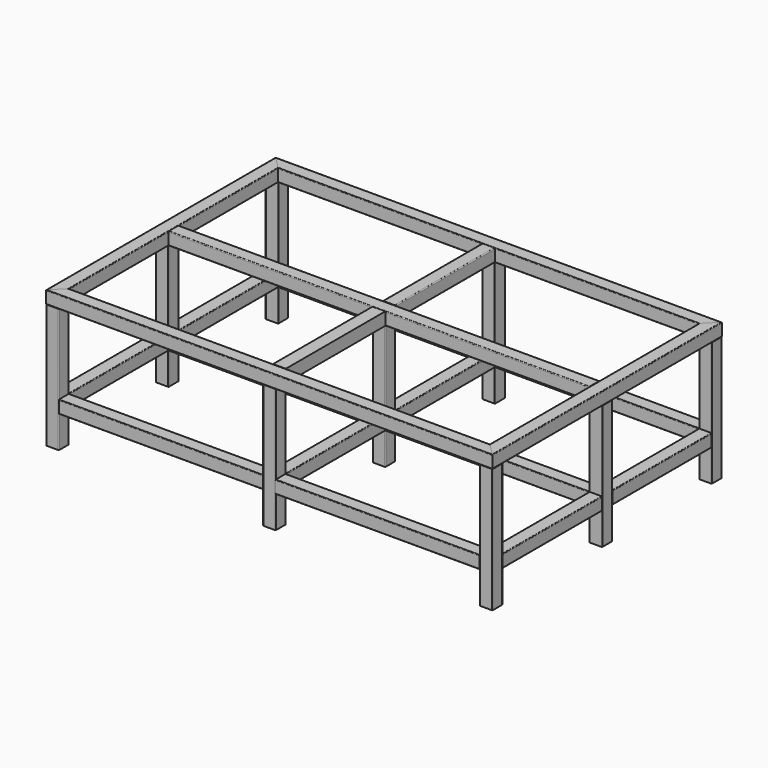
from build123d import *

# Parameters (mm, degrees)
F1_DEPTH  = 80
F2_W      = 70
F2_H      = 70
F3_DEPTH  = 1000
F4_R      = 4
F5_R      = 4
F7_DEPTH  = 80
F8_W      = 70
F8_H      = 70
F9_DEPTH  = 1400
F10_R     = 4
F11_R     = 4
F12_W     = 2640
F12_H     = 80
F13_DEPTH = 80
F14_W     = 70
F14_H     = 70
F15_DEPTH = 2640
F16_R     = 5
F17_W     = 80
F17_H     = 780
F18_DEPTH = 80
F19_W     = 70
F19_H     = 70
F20_DEPTH = 1560
F21_W     = 70
F21_H     = 70
F22_DEPTH = 1640
F23_R     = 5
F24_W     = 3000
F24_H     = 2000
F25_DEPTH = 60
F27_DEPTH = 780
F28_W     = 1280
F28_H     = 80
F29_DEPTH = 80
F31_DEPTH = 1280
F32_R     = 4
F34_DEPTH = 1280
F35_R     = 4
F36_W     = 1280
F36_H     = 80
F37_DEPTH = 80
F38_W     = 1280
F38_H     = 80
F39_DEPTH = 80
F41_DEPTH = 1280
F42_R     = 4
F42_2_R   = 4
F44_DEPTH = 1280
F45_R     = 4
F46_R     = 4
F47_W     = 780
F47_H     = 80
F48_DEPTH = 80
F49_W     = 780
F49_H     = 80
F50_DEPTH = 80
F51_W     = 780
F51_H     = 80
F52_DEPTH = 80
F54_DEPTH = 780
F55_R     = 4
F55_2_R   = 4
F55_3_R   = 4
F57_DEPTH = 780
F58_R     = 4
F58_2_R   = 4
F58_3_R   = 4


with BuildPart() as f1:
    # F0 (on Top) → F1 (new body)
    with BuildSketch(Plane.XY):
        Polygon((-1400, 900), (-1400, -900), (-1320, -820), (-1320, 820), align=None)
    extrude(amount=F1_DEPTH)


with BuildPart() as f1b:
    # F0 (on Top) → F1, piece 2 (new body)
    with BuildSketch(Plane.XY):
        Polygon((1320, 820), (1320, -820), (1400, -900), (1400, 900), align=None)
    extrude(amount=F1_DEPTH)


with BuildPart() as f3_tool:
    # F2 (on Front) → F3 (new body, symmetric)
    with BuildSketch(Plane.XZ):
        with Locations((-1360, 40)):
            Rectangle(F2_W, F2_H)
        with Locations((1360, 40)):
            Rectangle(F2_W, F2_H)
    extrude(amount=F3_DEPTH, both=True)


with BuildPart() as f1_1:
    add(f1.part)

    # F3: cut by f3_tool
    add(f3_tool.part, mode=Mode.SUBTRACT)

    # F4
    f4_edges = [f1_1.edges().sort_by_distance(p)[0] for p in [
        (-1400, 0, 80),
        (-1320, 0, 80),
        (-1320, 0, 0),
        (-1400, 0, 0),
        (-1325, 0, 75),
        (-1395, 0, 75),
        (-1325, 0, 5),
        (-1395, 0, 5),
    ]]
    fillet(f4_edges, radius=F4_R)


with BuildPart() as f1b_1:
    add(f1b.part)

    # F3: cut by f3_tool
    add(f3_tool.part, mode=Mode.SUBTRACT)

    # F5
    f5_edges = [f1b_1.edges().sort_by_distance(p)[0] for p in [
        (1400, 0, 80),
        (1400, 0, 0),
        (1320, 0, 80),
        (1320, 0, 0),
        (1395, 0, 75),
        (1395, 0, 5),
        (1325, 0, 5),
        (1325, 0, 75),
    ]]
    fillet(f5_edges, radius=F5_R)


with BuildPart() as f7:
    # F6 (on Top) → F7 (new body)
    with BuildSketch(Plane.XY):
        Polygon((1320, -820), (-1320, -820), (-1400, -900), (1400, -900), align=None)
    extrude(amount=F7_DEPTH)


with BuildPart() as f7b:
    # F6 (on Top) → F7, piece 2 (new body)
    with BuildSketch(Plane.XY):
        Polygon((1400, 900), (-1400, 900), (-1320, 820), (1320, 820), align=None)
    extrude(amount=F7_DEPTH)


with BuildPart() as f9_tool:
    # F8 (on Right) → F9 (new body, symmetric)
    with BuildSketch(Plane.YZ):
        with Locations((-860, 40)):
            Rectangle(F8_W, F8_H)
        with Locations((860, 40)):
            Rectangle(F8_W, F8_H)
    extrude(amount=F9_DEPTH, both=True)


with BuildPart() as f7_1:
    add(f7.part)

    # F9: cut by f9_tool
    add(f9_tool.part, mode=Mode.SUBTRACT)

    # F10
    f10_edges = [f7_1.edges().sort_by_distance(p)[0] for p in [
        (0, -900, 0),
        (0, -820, 0),
        (0, -820, 80),
        (0, -900, 80),
        (0, -895, 5),
        (0, -825, 5),
        (0, -825, 75),
        (0, -895, 75),
    ]]
    fillet(f10_edges, radius=F10_R)


with BuildPart() as f7b_1:
    add(f7b.part)

    # F9: cut by f9_tool
    add(f9_tool.part, mode=Mode.SUBTRACT)

    # F11
    f11_edges = [f7b_1.edges().sort_by_distance(p)[0] for p in [
        (0, 820, 80),
        (0, 900, 80),
        (0, 820, 0),
        (0, 895, 5),
        (0, 895, 75),
        (0, 900, 0),
        (0, 825, 75),
        (0, 825, 5),
    ]]
    fillet(f11_edges, radius=F11_R)


with BuildPart() as f13:
    # F12 (on Top) → F13 (new body)
    with BuildSketch(Plane.XY):
        Rectangle(F12_W, F12_H)
    extrude(amount=F13_DEPTH)

    # F14 (on face) → F15 (cut)
    with BuildSketch(Plane(origin=(-1320, 0, 0), x_dir=(0, -1, 0), z_dir=(-1, 0, 0))):
        with Locations((0, 40)):
            Rectangle(F14_W, F14_H)
    extrude(amount=-F15_DEPTH, mode=Mode.SUBTRACT)

    # F16
    f16_edges = [f13.edges().sort_by_distance(p)[0] for p in [
        (0, -40, 0),
        (0, 40, 0),
        (0, 40, 80),
        (0, -35, 75),
        (0, -40, 80),
        (0, -35, 5),
        (0, 35, 5),
        (0, 35, 75),
    ]]
    fillet(f16_edges, radius=F16_R)


with BuildPart() as f18:
    # F17 (on Top) → F18 (new body)
    with BuildSketch(Plane.XY):
        with Locations((0, 430)):
            Rectangle(F17_W, F17_H)
    extrude(amount=F18_DEPTH)


with BuildPart() as f18b:
    # F17 (on Top) → F18, piece 2 (new body)
    with BuildSketch(Plane.XY):
        with Locations((0, -430)):
            Rectangle(F17_W, F17_H)
    extrude(amount=F18_DEPTH)


with BuildPart() as f20_tool:
    # F19 (on face) → F20 (new body)
    with BuildSketch(Plane.XZ.offset(820)):
        with Locations((0, 40)):
            Rectangle(F19_W, F19_H)
    extrude(amount=-F20_DEPTH)


with BuildPart() as f18_1:
    add(f18.part)

    # F20: cut by f20_tool
    add(f20_tool.part, mode=Mode.SUBTRACT)

    # F21 (on face) → F22 (cut)
    with BuildSketch(Plane(origin=(0, 820, 0), x_dir=(-1, 0, 0), z_dir=(0, 1, 0))):
        with Locations((0, 40)):
            Rectangle(F21_W, F21_H)
    extrude(amount=-F22_DEPTH, mode=Mode.SUBTRACT)

    # F23
    f23_edges = [f18_1.edges().sort_by_distance(p)[0] for p in [
        (40, 430, 80),
        (-40, 430, 80),
        (40, 430, 0),
        (-40, 430, 0),
        (35, 430, 75),
        (35, 430, 5),
        (-35, 430, 5),
        (-35, 430, 75),
    ]]
    fillet(f23_edges, radius=F23_R)


with BuildPart() as f18b_1:
    add(f18b.part)

    # F20: cut by f20_tool
    add(f20_tool.part, mode=Mode.SUBTRACT)


with BuildPart() as f25:
    # F24 (on face) → F25 (new body)
    with BuildSketch(Plane.XY.offset(80)):
        Rectangle(F24_W, F24_H)
    extrude(amount=F25_DEPTH)


with BuildPart() as f27:
    # F26 (on face) → F27 (new body)
    with BuildSketch(Plane(origin=(0, 0, 0), x_dir=(1, 0, 0), z_dir=(0, 0, -1))):
        with BuildLine():
            Line((1324, -900), (1396, -900))
            ThreePointArc((1396, -900), (1398.8284271247, -898.8284271247), (1400, -896))
            Line((1400, -896), (1400, -824))
            ThreePointArc((1400, -824), (1398.8284271247, -821.1715728753), (1396, -820))
            Line((1396, -820), (1324, -820))
            ThreePointArc((1324, -820), (1321.1715728753, -821.1715728753), (1320, -824))
            Line((1320, -824), (1320, -896))
            ThreePointArc((1320, -896), (1321.1715728753, -898.8284271247), (1324, -900))
        make_face()
        with BuildLine():
            Line((1329, -825), (1391, -825))
            ThreePointArc((1391, -825), (1393.8284271247, -826.1715728753), (1395, -829))
            Line((1395, -829), (1395, -891))
            ThreePointArc((1395, -891), (1393.8284271247, -893.8284271247), (1391, -895))
            Line((1391, -895), (1329, -895))
            ThreePointArc((1329, -895), (1326.1715728753, -893.8284271247), (1325, -891))
            Line((1325, -891), (1325, -829))
            ThreePointArc((1325, -829), (1326.1715728753, -826.1715728753), (1329, -825))
        make_face(mode=Mode.SUBTRACT)
    extrude(amount=F27_DEPTH)


with BuildPart() as f27b:
    # F26 (on face) → F27, piece 2 (new body)
    with BuildSketch(Plane(origin=(0, 0, 0), x_dir=(1, 0, 0), z_dir=(0, 0, -1))):
        with BuildLine():
            ThreePointArc((1320, 824), (1321.1715728753, 821.1715728753), (1324, 820))
            Line((1324, 820), (1396, 820))
            ThreePointArc((1396, 820), (1398.8284271247, 821.1715728753), (1400, 824))
            Line((1400, 824), (1400, 896))
            ThreePointArc((1400, 896), (1398.8284271247, 898.8284271247), (1396, 900))
            Line((1396, 900), (1324, 900))
            ThreePointArc((1324, 900), (1321.1715728753, 898.8284271247), (1320, 896))
            Line((1320, 896), (1320, 824))
        make_face()
        with BuildLine():
            Line((1329, 895), (1391, 895))
            ThreePointArc((1391, 895), (1393.8284271247, 893.8284271247), (1395, 891))
            Line((1395, 891), (1395, 829))
            ThreePointArc((1395, 829), (1393.8284271247, 826.1715728753), (1391, 825))
            Line((1391, 825), (1329, 825))
            ThreePointArc((1329, 825), (1326.1715728753, 826.1715728753), (1325, 829))
            Line((1325, 829), (1325, 891))
            ThreePointArc((1325, 891), (1326.1715728753, 893.8284271247), (1329, 895))
        make_face(mode=Mode.SUBTRACT)
    extrude(amount=F27_DEPTH)


with BuildPart() as f27c:
    # F26 (on face) → F27, piece 3 (new body)
    with BuildSketch(Plane(origin=(0, 0, 0), x_dir=(1, 0, 0), z_dir=(0, 0, -1))):
        with BuildLine():
            ThreePointArc((-1396, 900), (-1398.8284271247, 898.8284271247), (-1400, 896))
            Line((-1400, 896), (-1400, 824))
            ThreePointArc((-1400, 824), (-1398.8284271247, 821.1715728753), (-1396, 820))
            Line((-1396, 820), (-1324, 820))
            ThreePointArc((-1324, 820), (-1321.1715728753, 821.1715728753), (-1320, 824))
            Line((-1320, 824), (-1320, 896))
            ThreePointArc((-1320, 896), (-1321.1715728753, 898.8284271247), (-1324, 900))
            Line((-1324, 900), (-1396, 900))
        make_face()
        with BuildLine():
            ThreePointArc((-1325, 829), (-1326.1715728753, 826.1715728753), (-1329, 825))
            Line((-1329, 825), (-1391, 825))
            ThreePointArc((-1391, 825), (-1393.8284271247, 826.1715728753), (-1395, 829))
            Line((-1395, 829), (-1395, 891))
            ThreePointArc((-1395, 891), (-1393.8284271247, 893.8284271247), (-1391, 895))
            Line((-1391, 895), (-1329, 895))
            ThreePointArc((-1329, 895), (-1326.1715728753, 893.8284271247), (-1325, 891))
            Line((-1325, 891), (-1325, 829))
        make_face(mode=Mode.SUBTRACT)
    extrude(amount=F27_DEPTH)


with BuildPart() as f27d:
    # F26 (on face) → F27, piece 4 (new body)
    with BuildSketch(Plane(origin=(0, 0, 0), x_dir=(1, 0, 0), z_dir=(0, 0, -1))):
        with BuildLine():
            ThreePointArc((-1320, -824), (-1321.1715728753, -821.1715728753), (-1324, -820))
            Line((-1324, -820), (-1396, -820))
            ThreePointArc((-1396, -820), (-1398.8284271247, -821.1715728753), (-1400, -824))
            Line((-1400, -824), (-1400, -896))
            ThreePointArc((-1400, -896), (-1398.8284271247, -898.8284271247), (-1396, -900))
            Line((-1396, -900), (-1324, -900))
            ThreePointArc((-1324, -900), (-1321.1715728753, -898.8284271247), (-1320, -896))
            Line((-1320, -896), (-1320, -824))
        make_face()
        with BuildLine():
            Line((-1391, -825), (-1329, -825))
            ThreePointArc((-1329, -825), (-1326.1715728753, -826.1715728753), (-1325, -829))
            Line((-1325, -829), (-1325, -891))
            ThreePointArc((-1325, -891), (-1326.1715728753, -893.8284271247), (-1329, -895))
            Line((-1329, -895), (-1391, -895))
            ThreePointArc((-1391, -895), (-1393.8284271247, -893.8284271247), (-1395, -891))
            Line((-1395, -891), (-1395, -829))
            ThreePointArc((-1395, -829), (-1393.8284271247, -826.1715728753), (-1391, -825))
        make_face(mode=Mode.SUBTRACT)
    extrude(amount=F27_DEPTH)


with BuildPart() as f27e:
    # F26 (on face) → F27, piece 5 (new body)
    with BuildSketch(Plane(origin=(0, 0, 0), x_dir=(1, 0, 0), z_dir=(0, 0, -1))):
        with BuildLine():
            ThreePointArc((40, -824), (38.8284271247, -821.1715728753), (36, -820))
            Line((36, -820), (-36, -820))
            ThreePointArc((-36, -820), (-38.8284271247, -821.1715728753), (-40, -824))
            Line((-40, -824), (-40, -896))
            ThreePointArc((-40, -896), (-38.8284271247, -898.8284271247), (-36, -900))
            Line((-36, -900), (36, -900))
            ThreePointArc((36, -900), (38.8284271247, -898.8284271247), (40, -896))
            Line((40, -896), (40, -824))
        make_face()
        with BuildLine():
            Line((-31, -825), (31, -825))
            ThreePointArc((31, -825), (33.8284271247, -826.1715728753), (35, -829))
            Line((35, -829), (35, -891))
            ThreePointArc((35, -891), (33.8284271247, -893.8284271247), (31, -895))
            Line((31, -895), (-31, -895))
            ThreePointArc((-31, -895), (-33.8284271247, -893.8284271247), (-35, -891))
            Line((-35, -891), (-35, -829))
            ThreePointArc((-35, -829), (-33.8284271247, -826.1715728753), (-31, -825))
        make_face(mode=Mode.SUBTRACT)
    extrude(amount=F27_DEPTH)


with BuildPart() as f27f:
    # F26 (on face) → F27, piece 6 (new body)
    with BuildSketch(Plane(origin=(0, 0, 0), x_dir=(1, 0, 0), z_dir=(0, 0, -1))):
        with BuildLine():
            ThreePointArc((40, 36), (38.8284271247, 38.8284271247), (36, 40))
            Line((36, 40), (-36, 40))
            ThreePointArc((-36, 40), (-38.8284271247, 38.8284271247), (-40, 36))
            Line((-40, 36), (-40, -36))
            ThreePointArc((-40, -36), (-38.8284271247, -38.8284271247), (-36, -40))
            Line((-36, -40), (36, -40))
            ThreePointArc((36, -40), (38.8284271247, -38.8284271247), (40, -36))
            Line((40, -36), (40, 36))
        make_face()
        with BuildLine():
            Line((-31, 35), (31, 35))
            ThreePointArc((31, 35), (33.8284271247, 33.8284271247), (35, 31))
            Line((35, 31), (35, -31))
            ThreePointArc((35, -31), (33.8284271247, -33.8284271247), (31, -35))
            Line((31, -35), (-31, -35))
            ThreePointArc((-31, -35), (-33.8284271247, -33.8284271247), (-35, -31))
            Line((-35, -31), (-35, 31))
            ThreePointArc((-35, 31), (-33.8284271247, 33.8284271247), (-31, 35))
        make_face(mode=Mode.SUBTRACT)
    extrude(amount=F27_DEPTH)


with BuildPart() as f27g:
    # F26 (on face) → F27, piece 7 (new body)
    with BuildSketch(Plane(origin=(0, 0, 0), x_dir=(1, 0, 0), z_dir=(0, 0, -1))):
        with BuildLine():
            ThreePointArc((1324, 40), (1321.1715728753, 38.8284271247), (1320, 36))
            Line((1320, 36), (1320, -36))
            ThreePointArc((1320, -36), (1321.1715728753, -38.8284271247), (1324, -40))
            Line((1324, -40), (1396, -40))
            ThreePointArc((1396, -40), (1398.8284271247, -38.8284271247), (1400, -36))
            Line((1400, -36), (1400, 36))
            ThreePointArc((1400, 36), (1398.8284271247, 38.8284271247), (1396, 40))
            Line((1396, 40), (1324, 40))
        make_face()
        with BuildLine():
            Line((1325, -31), (1325, 31))
            ThreePointArc((1325, 31), (1326.1715728753, 33.8284271247), (1329, 35))
            Line((1329, 35), (1391, 35))
            ThreePointArc((1391, 35), (1393.8284271247, 33.8284271247), (1395, 31))
            Line((1395, 31), (1395, -31))
            ThreePointArc((1395, -31), (1393.8284271247, -33.8284271247), (1391, -35))
            Line((1391, -35), (1329, -35))
            ThreePointArc((1329, -35), (1326.1715728753, -33.8284271247), (1325, -31))
        make_face(mode=Mode.SUBTRACT)
    extrude(amount=F27_DEPTH)


with BuildPart() as f27h:
    # F26 (on face) → F27, piece 8 (new body)
    with BuildSketch(Plane(origin=(0, 0, 0), x_dir=(1, 0, 0), z_dir=(0, 0, -1))):
        with BuildLine():
            Line((-1324, 40), (-1396, 40))
            ThreePointArc((-1396, 40), (-1398.8284271247, 38.8284271247), (-1400, 36))
            Line((-1400, 36), (-1400, -36))
            ThreePointArc((-1400, -36), (-1398.8284271247, -38.8284271247), (-1396, -40))
            Line((-1396, -40), (-1324, -40))
            ThreePointArc((-1324, -40), (-1321.1715728753, -38.8284271247), (-1320, -36))
            Line((-1320, -36), (-1320, 36))
            ThreePointArc((-1320, 36), (-1321.1715728753, 38.8284271247), (-1324, 40))
        make_face()
        with BuildLine():
            ThreePointArc((-1395, 31), (-1393.8284271247, 33.8284271247), (-1391, 35))
            Line((-1391, 35), (-1329, 35))
            ThreePointArc((-1329, 35), (-1326.1715728753, 33.8284271247), (-1325, 31))
            Line((-1325, 31), (-1325, -31))
            ThreePointArc((-1325, -31), (-1326.1715728753, -33.8284271247), (-1329, -35))
            Line((-1329, -35), (-1391, -35))
            ThreePointArc((-1391, -35), (-1393.8284271247, -33.8284271247), (-1395, -31))
            Line((-1395, -31), (-1395, 31))
        make_face(mode=Mode.SUBTRACT)
    extrude(amount=F27_DEPTH)


with BuildPart() as f27i:
    # F26 (on face) → F27, piece 9 (new body)
    with BuildSketch(Plane(origin=(0, 0, 0), x_dir=(1, 0, 0), z_dir=(0, 0, -1))):
        with BuildLine():
            ThreePointArc((-36, 900), (-38.8284271247, 898.8284271247), (-40, 896))
            Line((-40, 896), (-40, 824))
            ThreePointArc((-40, 824), (-38.8284271247, 821.1715728753), (-36, 820))
            Line((-36, 820), (36, 820))
            ThreePointArc((36, 820), (38.8284271247, 821.1715728753), (40, 824))
            Line((40, 824), (40, 896))
            ThreePointArc((40, 896), (38.8284271247, 898.8284271247), (36, 900))
            Line((36, 900), (-36, 900))
        make_face()
        with BuildLine():
            ThreePointArc((-31, 825), (-33.8284271247, 826.1715728753), (-35, 829))
            Line((-35, 829), (-35, 891))
            ThreePointArc((-35, 891), (-33.8284271247, 893.8284271247), (-31, 895))
            Line((-31, 895), (31, 895))
            ThreePointArc((31, 895), (33.8284271247, 893.8284271247), (35, 891))
            Line((35, 891), (35, 829))
            ThreePointArc((35, 829), (33.8284271247, 826.1715728753), (31, 825))
            Line((31, 825), (-31, 825))
        make_face(mode=Mode.SUBTRACT)
    extrude(amount=F27_DEPTH)


with BuildPart() as f29:
    # F28 (on face) → F29 (new body)
    with BuildSketch(Plane.XZ.offset(900)):
        with Locations((-680, -540)):
            Rectangle(F28_W, F28_H)
    extrude(amount=-F29_DEPTH)

    # F33 (on face) → F34 (cut)
    with BuildSketch(Plane.YZ.offset(-40)):
        with BuildLine():
            Line((-829, -505), (-891, -505))
            ThreePointArc((-891, -505), (-893.8284271247, -506.1715728753), (-895, -509))
            Line((-895, -509), (-895, -571))
            ThreePointArc((-895, -571), (-893.8284271247, -573.8284271247), (-891, -575))
            Line((-891, -575), (-829, -575))
            ThreePointArc((-829, -575), (-826.1715728753, -573.8284271247), (-825, -571))
            Line((-825, -571), (-825, -509))
            ThreePointArc((-825, -509), (-826.1715728753, -506.1715728753), (-829, -505))
        make_face()
    extrude(amount=-F34_DEPTH, mode=Mode.SUBTRACT)

    # F35
    f35_edges = [f29.edges().sort_by_distance(p)[0] for p in [
        (-680, -900, -500),
        (-680, -820, -500),
        (-680, -900, -580),
        (-680, -820, -580),
    ]]
    fillet(f35_edges, radius=F35_R)


with BuildPart() as f29b:
    # F28 (on face) → F29, piece 2 (new body)
    with BuildSketch(Plane.XZ.offset(900)):
        with Locations((680, -540)):
            Rectangle(F28_W, F28_H)
    extrude(amount=-F29_DEPTH)

    # F30 (on face) → F31 (cut)
    with BuildSketch(Plane.YZ.offset(1320)):
        with BuildLine():
            Line((-829, -505), (-891, -505))
            ThreePointArc((-891, -505), (-893.8284271247, -506.1715728753), (-895, -509))
            Line((-895, -509), (-895, -571))
            ThreePointArc((-895, -571), (-893.8284271247, -573.8284271247), (-891, -575))
            Line((-891, -575), (-829, -575))
            ThreePointArc((-829, -575), (-826.1715728753, -573.8284271247), (-825, -571))
            Line((-825, -571), (-825, -509))
            ThreePointArc((-825, -509), (-826.1715728753, -506.1715728753), (-829, -505))
        make_face()
    extrude(amount=-F31_DEPTH, mode=Mode.SUBTRACT)

    # F32
    f32_edges = [f29b.edges().sort_by_distance(p)[0] for p in [
        (680, -900, -500),
        (680, -900, -580),
        (680, -820, -500),
        (680, -820, -580),
    ]]
    fillet(f32_edges, radius=F32_R)


with BuildPart() as f37:
    # F36 (on face) → F37 (new body)
    with BuildSketch(Plane.XZ.offset(40)):
        with Locations((-680, -540)):
            Rectangle(F36_W, F36_H)
    extrude(amount=-F37_DEPTH)


with BuildPart() as f37b:
    # F36 (on face) → F37, piece 2 (new body)
    with BuildSketch(Plane.XZ.offset(40)):
        with Locations((680, -540)):
            Rectangle(F36_W, F36_H)
    extrude(amount=-F37_DEPTH)


with BuildPart() as f39:
    # F38 (on face) → F39 (new body)
    with BuildSketch(Plane(origin=(0, 900, 0), x_dir=(-1, 0, 0), z_dir=(0, 1, 0))):
        with Locations((-680, -540)):
            Rectangle(F38_W, F38_H)
    extrude(amount=-F39_DEPTH)


with BuildPart() as f39b:
    # F38 (on face) → F39, piece 2 (new body)
    with BuildSketch(Plane(origin=(0, 900, 0), x_dir=(-1, 0, 0), z_dir=(0, 1, 0))):
        with Locations((680, -540)):
            Rectangle(F38_W, F38_H)
    extrude(amount=-F39_DEPTH)


with BuildPart() as f41_tool:
    # F40 (on face) → F41 (new body)
    with BuildSketch(Plane.YZ.offset(1320)):
        with BuildLine():
            Line((31, -505), (-31, -505))
            ThreePointArc((-31, -505), (-33.8284271247, -506.1715728753), (-35, -509))
            Line((-35, -509), (-35, -571))
            ThreePointArc((-35, -571), (-33.8284271247, -573.8284271247), (-31, -575))
            Line((-31, -575), (31, -575))
            ThreePointArc((31, -575), (33.8284271247, -573.8284271247), (35, -571))
            Line((35, -571), (35, -509))
            ThreePointArc((35, -509), (33.8284271247, -506.1715728753), (31, -505))
        make_face()
        with BuildLine():
            Line((891, -505), (829, -505))
            ThreePointArc((829, -505), (826.1715728753, -506.1715728753), (825, -509))
            Line((825, -509), (825, -571))
            ThreePointArc((825, -571), (826.1715728753, -573.8284271247), (829, -575))
            Line((829, -575), (891, -575))
            ThreePointArc((891, -575), (893.8284271247, -573.8284271247), (895, -571))
            Line((895, -571), (895, -509))
            ThreePointArc((895, -509), (893.8284271247, -506.1715728753), (891, -505))
        make_face()
    extrude(amount=-F41_DEPTH)


with BuildPart() as f37b_1:
    add(f37b.part)

    # F41: cut by f41_tool
    add(f41_tool.part, mode=Mode.SUBTRACT)

    # F42
    f42_edges = [f37b_1.edges().sort_by_distance(p)[0] for p in [
        (680, -40, -500),
        (680, 40, -500),
        (680, -40, -580),
        (680, 40, -580),
    ]]
    fillet(f42_edges, radius=F42_R)


with BuildPart() as f39_1:
    add(f39.part)

    # F41: cut by f41_tool
    add(f41_tool.part, mode=Mode.SUBTRACT)

    # F42#2
    f42_2_edges = [f39_1.edges().sort_by_distance(p)[0] for p in [
        (680, 900, -580),
        (680, 900, -500),
        (680, 820, -500),
        (680, 820, -580),
    ]]
    fillet(f42_2_edges, radius=F42_2_R)


with BuildPart() as f44_tool:
    # F43 (on face) → F44 (new body)
    with BuildSketch(Plane(origin=(-1320, 0, 0), x_dir=(0, -1, 0), z_dir=(-1, 0, 0))):
        with BuildLine():
            Line((-829, -505), (-891, -505))
            ThreePointArc((-891, -505), (-893.8284271247, -506.1715728753), (-895, -509))
            Line((-895, -509), (-895, -571))
            ThreePointArc((-895, -571), (-893.8284271247, -573.8284271247), (-891, -575))
            Line((-891, -575), (-829, -575))
            ThreePointArc((-829, -575), (-826.1715728753, -573.8284271247), (-825, -571))
            Line((-825, -571), (-825, -509))
            ThreePointArc((-825, -509), (-826.1715728753, -506.1715728753), (-829, -505))
        make_face()
        with BuildLine():
            Line((31, -505), (-31, -505))
            ThreePointArc((-31, -505), (-33.8284271247, -506.1715728753), (-35, -509))
            Line((-35, -509), (-35, -571))
            ThreePointArc((-35, -571), (-33.8284271247, -573.8284271247), (-31, -575))
            Line((-31, -575), (31, -575))
            ThreePointArc((31, -575), (33.8284271247, -573.8284271247), (35, -571))
            Line((35, -571), (35, -509))
            ThreePointArc((35, -509), (33.8284271247, -506.1715728753), (31, -505))
        make_face()
    extrude(amount=-F44_DEPTH)


with BuildPart() as f37_1:
    add(f37.part)

    # F44: cut by f44_tool
    add(f44_tool.part, mode=Mode.SUBTRACT)

    # F46
    f46_edges = [f37_1.edges().sort_by_distance(p)[0] for p in [
        (-680, 40, -500),
        (-680, -40, -500),
        (-680, -40, -580),
        (-680, 40, -580),
    ]]
    fillet(f46_edges, radius=F46_R)


with BuildPart() as f39b_1:
    add(f39b.part)

    # F44: cut by f44_tool
    add(f44_tool.part, mode=Mode.SUBTRACT)

    # F45
    f45_edges = [f39b_1.edges().sort_by_distance(p)[0] for p in [
        (-680, 900, -500),
        (-680, 820, -500),
        (-680, 900, -580),
        (-680, 820, -580),
    ]]
    fillet(f45_edges, radius=F45_R)


with BuildPart() as f48:
    # F47 (on face) → F48 (new body)
    with BuildSketch(Plane.YZ.offset(1400)):
        with Locations((-430, -540)):
            Rectangle(F47_W, F47_H)
    extrude(amount=-F48_DEPTH)


with BuildPart() as f48b:
    # F47 (on face) → F48, piece 2 (new body)
    with BuildSketch(Plane.YZ.offset(1400)):
        with Locations((430, -540)):
            Rectangle(F47_W, F47_H)
    extrude(amount=-F48_DEPTH)


with BuildPart() as f50:
    # F49 (on face) → F50 (new body)
    with BuildSketch(Plane(origin=(-40, 0, 0), x_dir=(0, -1, 0), z_dir=(-1, 0, 0))):
        with Locations((-430, -540)):
            Rectangle(F49_W, F49_H)
    extrude(amount=-F50_DEPTH)


with BuildPart() as f50b:
    # F49 (on face) → F50, piece 2 (new body)
    with BuildSketch(Plane(origin=(-40, 0, 0), x_dir=(0, -1, 0), z_dir=(-1, 0, 0))):
        with Locations((430, -540)):
            Rectangle(F49_W, F49_H)
    extrude(amount=-F50_DEPTH)


with BuildPart() as f52:
    # F51 (on face) → F52 (new body)
    with BuildSketch(Plane(origin=(-1400, 0, 0), x_dir=(0, -1, 0), z_dir=(-1, 0, 0))):
        with Locations((-430, -540)):
            Rectangle(F51_W, F51_H)
    extrude(amount=-F52_DEPTH)


with BuildPart() as f52b:
    # F51 (on face) → F52, piece 2 (new body)
    with BuildSketch(Plane(origin=(-1400, 0, 0), x_dir=(0, -1, 0), z_dir=(-1, 0, 0))):
        with Locations((430, -540)):
            Rectangle(F51_W, F51_H)
    extrude(amount=-F52_DEPTH)


with BuildPart() as f54_tool:
    # F53 (on face) → F54 (new body)
    with BuildSketch(Plane(origin=(0, 820, 0), x_dir=(-1, 0, 0), z_dir=(0, 1, 0))):
        with BuildLine():
            Line((-1329, -505), (-1391, -505))
            ThreePointArc((-1391, -505), (-1393.8284271247, -506.1715728753), (-1395, -509))
            Line((-1395, -509), (-1395, -571))
            ThreePointArc((-1395, -571), (-1393.8284271247, -573.8284271247), (-1391, -575))
            Line((-1391, -575), (-1329, -575))
            ThreePointArc((-1329, -575), (-1326.1715728753, -573.8284271247), (-1325, -571))
            Line((-1325, -571), (-1325, -509))
            ThreePointArc((-1325, -509), (-1326.1715728753, -506.1715728753), (-1329, -505))
        make_face()
        with BuildLine():
            Line((31, -505), (-31, -505))
            ThreePointArc((-31, -505), (-33.8284271247, -506.1715728753), (-35, -509))
            Line((-35, -509), (-35, -571))
            ThreePointArc((-35, -571), (-33.8284271247, -573.8284271247), (-31, -575))
            Line((-31, -575), (31, -575))
            ThreePointArc((31, -575), (33.8284271247, -573.8284271247), (35, -571))
            Line((35, -571), (35, -509))
            ThreePointArc((35, -509), (33.8284271247, -506.1715728753), (31, -505))
        make_face()
        with BuildLine():
            Line((1391, -505), (1329, -505))
            ThreePointArc((1329, -505), (1326.1715728753, -506.1715728753), (1325, -509))
            Line((1325, -509), (1325, -571))
            ThreePointArc((1325, -571), (1326.1715728753, -573.8284271247), (1329, -575))
            Line((1329, -575), (1391, -575))
            ThreePointArc((1391, -575), (1393.8284271247, -573.8284271247), (1395, -571))
            Line((1395, -571), (1395, -509))
            ThreePointArc((1395, -509), (1393.8284271247, -506.1715728753), (1391, -505))
        make_face()
    extrude(amount=-F54_DEPTH)


with BuildPart() as f48b_1:
    add(f48b.part)

    # F54: cut by f54_tool
    add(f54_tool.part, mode=Mode.SUBTRACT)

    # F55
    f55_edges = [f48b_1.edges().sort_by_distance(p)[0] for p in [
        (1400, 430, -500),
        (1400, 430, -580),
        (1320, 430, -500),
        (1320, 430, -580),
    ]]
    fillet(f55_edges, radius=F55_R)


with BuildPart() as f50_1:
    add(f50.part)

    # F54: cut by f54_tool
    add(f54_tool.part, mode=Mode.SUBTRACT)

    # F55#2
    f55_2_edges = [f50_1.edges().sort_by_distance(p)[0] for p in [
        (40, 430, -580),
        (-40, 430, -580),
        (-40, 430, -500),
        (40, 430, -500),
    ]]
    fillet(f55_2_edges, radius=F55_2_R)


with BuildPart() as f52_1:
    add(f52.part)

    # F54: cut by f54_tool
    add(f54_tool.part, mode=Mode.SUBTRACT)

    # F55#3
    f55_3_edges = [f52_1.edges().sort_by_distance(p)[0] for p in [
        (-1400, 430, -500),
        (-1400, 430, -580),
        (-1320, 430, -580),
        (-1320, 430, -500),
    ]]
    fillet(f55_3_edges, radius=F55_3_R)


with BuildPart() as f57_tool:
    # F56 (on face) → F57 (new body)
    with BuildSketch(Plane.XZ.offset(820)):
        with BuildLine():
            Line((-1329, -505), (-1391, -505))
            ThreePointArc((-1391, -505), (-1393.8284271247, -506.1715728753), (-1395, -509))
            Line((-1395, -509), (-1395, -571))
            ThreePointArc((-1395, -571), (-1393.8284271247, -573.8284271247), (-1391, -575))
            Line((-1391, -575), (-1329, -575))
            ThreePointArc((-1329, -575), (-1326.1715728753, -573.8284271247), (-1325, -571))
            Line((-1325, -571), (-1325, -509))
            ThreePointArc((-1325, -509), (-1326.1715728753, -506.1715728753), (-1329, -505))
        make_face()
        with BuildLine():
            Line((31, -505), (-31, -505))
            ThreePointArc((-31, -505), (-33.8284271247, -506.1715728753), (-35, -509))
            Line((-35, -509), (-35, -571))
            ThreePointArc((-35, -571), (-33.8284271247, -573.8284271247), (-31, -575))
            Line((-31, -575), (31, -575))
            ThreePointArc((31, -575), (33.8284271247, -573.8284271247), (35, -571))
            Line((35, -571), (35, -509))
            ThreePointArc((35, -509), (33.8284271247, -506.1715728753), (31, -505))
        make_face()
        with BuildLine():
            Line((1391, -505), (1329, -505))
            ThreePointArc((1329, -505), (1326.1715728753, -506.1715728753), (1325, -509))
            Line((1325, -509), (1325, -571))
            ThreePointArc((1325, -571), (1326.1715728753, -573.8284271247), (1329, -575))
            Line((1329, -575), (1391, -575))
            ThreePointArc((1391, -575), (1393.8284271247, -573.8284271247), (1395, -571))
            Line((1395, -571), (1395, -509))
            ThreePointArc((1395, -509), (1393.8284271247, -506.1715728753), (1391, -505))
        make_face()
    extrude(amount=-F57_DEPTH)


with BuildPart() as f48_1:
    add(f48.part)

    # F57: cut by f57_tool
    add(f57_tool.part, mode=Mode.SUBTRACT)

    # F58
    f58_edges = [f48_1.edges().sort_by_distance(p)[0] for p in [
        (1400, -430, -580),
        (1320, -430, -580),
        (1400, -430, -500),
        (1320, -430, -500),
    ]]
    fillet(f58_edges, radius=F58_R)


with BuildPart() as f50b_1:
    add(f50b.part)

    # F57: cut by f57_tool
    add(f57_tool.part, mode=Mode.SUBTRACT)

    # F58#2
    f58_2_edges = [f50b_1.edges().sort_by_distance(p)[0] for p in [
        (40, -430, -580),
        (-40, -430, -580),
        (40, -430, -500),
        (-40, -430, -500),
    ]]
    fillet(f58_2_edges, radius=F58_2_R)


with BuildPart() as f52b_1:
    add(f52b.part)

    # F57: cut by f57_tool
    add(f57_tool.part, mode=Mode.SUBTRACT)

    # F58#3
    f58_3_edges = [f52b_1.edges().sort_by_distance(p)[0] for p in [
        (-1400, -430, -580),
        (-1400, -430, -500),
        (-1320, -430, -500),
        (-1320, -430, -580),
    ]]
    fillet(f58_3_edges, radius=F58_3_R)


solid = Compound([f1_1.part, f1b_1.part, f7_1.part, f7b_1.part, f13.part, f18_1.part, f18b_1.part, f27.part, f27b.part, f27c.part, f27d.part, f27e.part, f27f.part, f27g.part, f27h.part, f27i.part, f29.part, f29b.part, f37b_1.part, f39_1.part, f37_1.part, f39b_1.part, f48b_1.part, f50_1.part, f52_1.part, f48_1.part, f50b_1.part, f52b_1.part])
